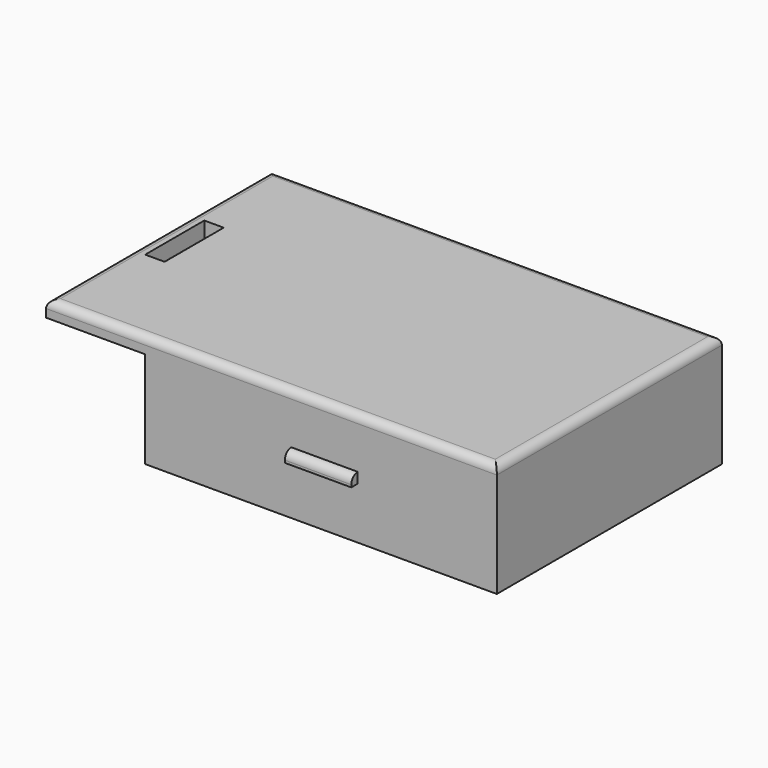
from build123d import *

# Parameters (mm, degrees)
F0_W     = 142.1354152262
F0_H     = 88.716968894
F1_DEPTH = 5.08
F2_W     = 6.1184130609
F2_H     = 23.2970286161
F3_DEPTH = 25.4
F4_W     = 110.9326332808
F4_H     = 88.716968894
F5_DEPTH = 30.48
F6_W     = 20.9437925369
F6_H     = 3.2945293933
F7_DEPTH = 2.54
F8_R     = 2.54
F9_R     = 2.53999


# Not quite as in the source:
# - a fillet or chamfer is up to 0.001 mm smaller than in the source, because OpenCascade refuses the exact size


with BuildPart() as f1:
    # F0 (on Top) → F1 (new body)
    with BuildSketch(Plane.XY):
        with Locations((16.7079698294, 10.4718953371)):
            Rectangle(F0_W, F0_H)
    extrude(amount=F1_DEPTH)

    # F2 (on face) → F3 (cut)
    with BuildSketch(Plane.XY.offset(5.08)):
        with Locations((-47.1599567682, 11.648514308)):
            Rectangle(F2_W, F2_H)
    extrude(amount=-F3_DEPTH, mode=Mode.SUBTRACT)

    # F4 (on face) → F5 (join)
    with BuildSketch(Plane(origin=(0, 0, 0), x_dir=(1, 0, 0), z_dir=(0, 0, -1))):
        with Locations((32.3093608022, -10.4718953371)):
            Rectangle(F4_W, F4_H)
    extrude(amount=F5_DEPTH)

    # F6 (on face) → F7 (join)
    with BuildSketch(Plane.XZ.offset(33.8865891099)):
        with Locations((33.4383537993, -12.4721480533)):
            Rectangle(F6_W, F6_H)
    extrude(amount=F7_DEPTH)

    # F8
    f8_edges = [f1.edges().sort_by_distance(p)[0] for p in [
        (16.70797, -33.886589, 5.08),
        (-54.359738, 10.471895, 5.08),
        (16.70797, 54.83038, 5.08),
        (87.775677, 10.471895, 5.08),
    ]]
    fillet(f8_edges, radius=F8_R)

    # F9 (radius 2.54 in the source; OpenCascade refuses exactly that, so slightly less here)
    f9_edges = [f1.edges().sort_by_distance(p)[0] for p in [
        (33.438354, -36.426589, -10.824883),
    ]]
    fillet(f9_edges, radius=F9_R)


solid = f1.part
